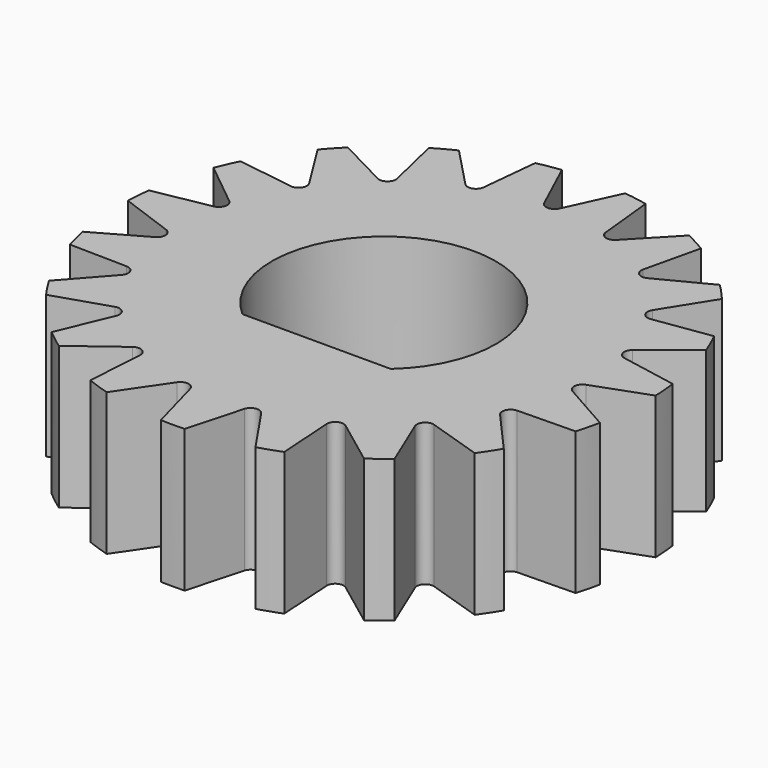
from build123d import *

# Parameters (mm, degrees)
F0_R            = 9.4221007419
F1_DEPTH        = 5.08
F3_DEPTH        = 5.08
F3_COPIES_COUNT = 19


# Not quite as in the source:
# - a pattern or mirror of a feature is missing from the dataset's text; its kind, count and spacing are read off the source's solid
# - a feature names something its author has since deleted; it is built from what else it names


with BuildPart() as f1:
    # F0 (on Top) → F1 (new body)
    with BuildSketch(Plane.XY):
        Circle(F0_R)
        with BuildLine():
            ThreePointArc((-2.6457529, -2.9999985987), (0, 4), (2.6457529, -2.9999985987))
            Line((2.6457529, -2.9999985987), (-2.6457529, -2.9999985987))
        make_face(mode=Mode.SUBTRACT)
    extrude(amount=F1_DEPTH)

    # F2 (on face) → F3 (cut, through all)
    with BuildSketch(Plane.XY.offset(5.08)):
        with BuildLine():
            Line((0.2702110818, 7.4907975301), (1.1292079793, 9.3541900628))
            ThreePointArc((1.1292079793, 9.3541900628), (0, 9.4221007419), (-1.1292079793, 9.3541900628))
            Line((-1.1292079793, 9.3541900628), (-0.2702110818, 7.4907975301))
            ThreePointArc((-0.2702110818, 7.4907975301), (0, 7.3178208914), (0.2702110818, 7.4907975301))
        make_face()
    f3 = extrude(amount=-F3_DEPTH, mode=Mode.SUBTRACT)

    # F3_copies: F3 ×19 about axis
    f3_copies_axis = Axis((0, 0, 0), (0, 0, 1))
    for i in range(1, F3_COPIES_COUNT):
        add(f3.rotate(f3_copies_axis, i * 360 / F3_COPIES_COUNT), mode=Mode.SUBTRACT)


solid = f1.part
